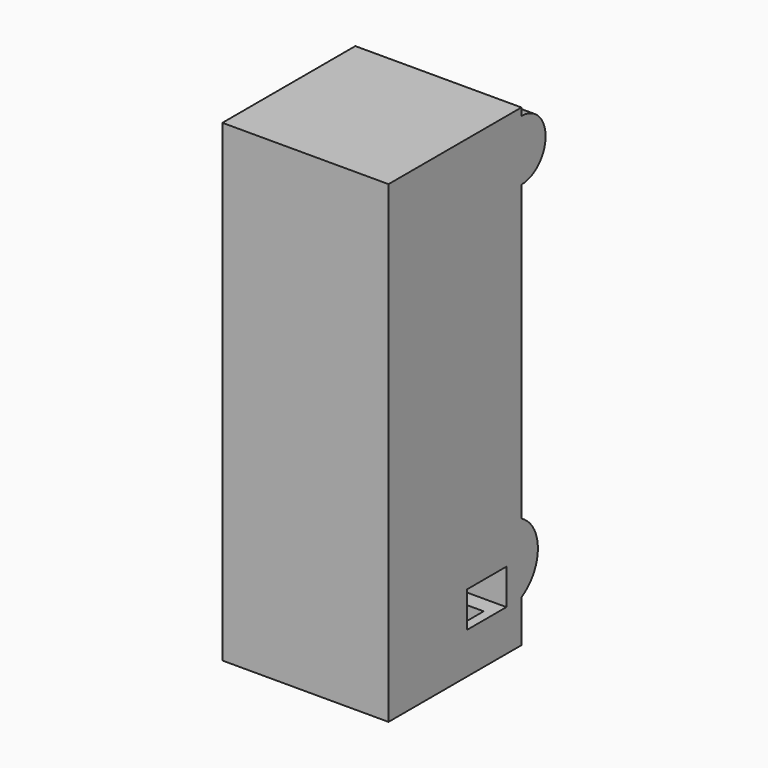
from build123d import *

# Parameters (mm, degrees)
F0_W        = 100
F0_H        = 100
F1_DEPTH    = 100
F2_W        = 88.9338813722
F2_H        = 88.2601328194
F3_DEPTH    = 90
F5_DEPTH    = 185
F6_T        = 5
F6_T3_DEPTH = 100
F6_T5_DEPTH = 98.2601328194
F6_T7_DEPTH = 98.9338813722
F7_W        = 90
F7_H        = 95
F8_DEPTH    = 8
F10_DEPTH   = 25
F11_R       = 23.6849070482
F11_R_2     = 18.1970048193
F12_DEPTH   = 25
F13_W       = 74.0287862718
F13_H       = 40.3192453086
F14_DEPTH   = 9
F15_W       = 33.1602711231
F15_H       = 63.8056004047
F16_DEPTH   = 25
F17_W       = 95
F17_H       = 277
F18_DEPTH   = 31
F19_W       = 29.5484475791
F19_H       = 21.4659199119
F20_DEPTH   = 25


# Not quite as in the source:
# - a shell that OpenCascade refuses in one call is made with other operations: the cavity is built on its own and cut out


with BuildPart() as f1:
    # F0 (on Front) → F1 (new body)
    with BuildSketch(Plane.XZ):
        with Locations((-6.5152887255, 3.7536189136)):
            Rectangle(F0_W, F0_H)
    extrude(amount=F1_DEPTH)

    # F2 (on face) → F3 (cut)
    with BuildSketch(Plane.XZ.offset(100)):
        with Locations((-6.6661592573, 4.4211242348)):
            Rectangle(F2_W, F2_H)
    extrude(amount=-F3_DEPTH, mode=Mode.SUBTRACT)

    # F4 (on face) → F5 (join)
    with BuildSketch(Plane.XY.offset(53.7536189136)):
        Polygon((-56.5152887255, -100), (43.4847112745, -100), (43.4847112745, -33.4126986563), (43.4847112745, 0), (-56.5152887255, 0), align=None)
    extrude(amount=F5_DEPTH)

    # F6: shell of thickness 5, made by hand


with BuildPart() as f6_core1:
    # F6_t2: copy of F1
    add(f1.part)

    # the walls: a layer under each face that stays
    f6_faces = [f6_core1.faces().sort_by_distance(p)[0] for p in [
        (43.4847112745, -50, 96.2536189136),
        (-6.5152887255, 0, 96.2536189136),
        (-56.5152887255, -50, 96.2536189136),
        (-51.1330999434, -55, 4.4211242348),
        (-6.6661592573, -10, 4.4211242348),
        (-6.6661592573, -55, -39.7089421749),
        (37.8007814288, -55, 4.4211242348),
        (-6.6661592573, -55, 48.5511906445),
        (-6.5152887255, -50, -46.2463810864),
    ]]
    thicken(f6_faces, amount=-F6_T, mode=Mode.SUBTRACT)

    # F6_s4 → F6_t3 (cut)
    with BuildSketch(Plane.XZ.offset(5)):
        Polygon((-51.0830999434, 48.5011906445), (-56.1330999434, 48.5511906445), (-56.1330999434, 53.5511906445), (-51.1330999434, 53.5511906445), align=None)
        Polygon((-51.0830999434, -39.6589421749), (-56.1330999434, -39.7089421749), (-56.1330999434, -44.7089421749), (-51.1330999434, -44.7089421749), align=None)
        Polygon((37.7507814288, -39.6589421749), (37.8007814288, -44.7089421749), (42.8007814288, -44.7089421749), (42.8007814288, -39.7089421749), align=None)
        Polygon((37.7507814288, 48.5011906445), (42.8007814288, 48.5511906445), (42.8007814288, 53.5511906445), (37.8007814288, 53.5511906445), align=None)
    extrude(amount=F6_T3_DEPTH, mode=Mode.SUBTRACT)

    # F6_s6 → F6_t5 (cut)
    with BuildSketch(Plane.XY.offset(-44.7089421749)):
        Polygon((-51.0830999434, -10.05), (-56.1330999434, -10), (-56.1330999434, -5), (-51.1330999434, -5), align=None)
        Polygon((37.7507814288, -10.05), (37.8007814288, -5), (42.8007814288, -5), (42.8007814288, -10), align=None)
    extrude(amount=F6_T5_DEPTH, mode=Mode.SUBTRACT)

    # F6_s8 → F6_t7 (cut)
    with BuildSketch(Plane.YZ.offset(-56.1330999434)):
        Polygon((-10.05, 48.5011906445), (-5, 48.5511906445), (-5, 53.5511906445), (-10, 53.5511906445), align=None)
        Polygon((-10.05, -39.6589421749), (-5, -39.7089421749), (-5, -44.7089421749), (-10, -44.7089421749), align=None)
    extrude(amount=F6_T7_DEPTH, mode=Mode.SUBTRACT)


with BuildPart() as f1_1:
    add(f1.part)

    # what is left inside the walls is the cavity
    f6_cavity = [f6_core1.part.solids().sort_by_distance(p)[0] for p in [
        (38.434711, -68.333333, 146.152405),
    ]]
    add(f6_cavity, mode=Mode.SUBTRACT)

    # F7 (on face) → F8 (join)
    with BuildSketch(Plane.XY.offset(238.7536189136)):
        with Locations((-6.5152887255, -52.5)):
            Rectangle(F7_W, F7_H)
    extrude(amount=-F8_DEPTH)

    # F9 (on face) → F10 (join)
    with BuildSketch(Plane(origin=(-56.5152887255, 0, 0), x_dir=(0, -1, 0), z_dir=(-1, 0, 0))):
        with BuildLine():
            ThreePointArc((0, 189.510354193), (12.2569085004, 194.5873319266), (17.333886234, 206.844240427))
            ThreePointArc((17.333886234, 206.844240427), (12.2569085004, 219.1011489274), (0, 224.178126661))
            Line((0, 224.178126661), (0, 189.510354193))
        make_face()
        with BuildLine():
            Line((0, 189.510354193), (0, 224.178126661))
            ThreePointArc((0, 224.178126661), (-17.333886234, 206.844240427), (0, 189.510354193))
        make_face()
        with BuildLine():
            Line((0, -23.6541135693), (0, 23.6541135693))
            ThreePointArc((0, 23.6541135693), (-15.7209434523, 0), (0, -23.6541135693))
        make_face()
    extrude(amount=-F10_DEPTH)

    # F11 (on face) → F12 (join)
    with BuildSketch(Plane.YZ.offset(43.4847112745)):
        with Locations((-11.2718828022, 0)):
            Circle(F11_R)
        with Locations((0, 216.0427719355)):
            Circle(F11_R_2)
    extrude(amount=-F12_DEPTH)

    # F13 (on face) → F14 (cut)
    with BuildSketch(Plane(origin=(0, 0, -46.2463810864), x_dir=(1, 0, 0), z_dir=(0, 0, -1))):
        with Locations((-6.1139781028, 59.594200924)):
            Rectangle(F13_W, F13_H)
    extrude(amount=-F14_DEPTH, mode=Mode.SUBTRACT)

    # F15 (on face) → F16 (cut)
    with BuildSketch(Plane(origin=(0, 0, 48.5511906445), x_dir=(1, 0, 0), z_dir=(0, 0, -1))):
        with Locations((9.9139763042, 41.9028002024)):
            Rectangle(F15_W, F15_H)
    extrude(amount=-F16_DEPTH, mode=Mode.SUBTRACT)

    # F17 (on face) → F18 (join)
    with BuildSketch(Plane.XZ.offset(100)):
        with Locations((-9.0152887255, 92.2536189136)):
            Rectangle(F17_W, F17_H)
    extrude(amount=-F18_DEPTH)

    # F19 (on face) → F20 (cut)
    with BuildSketch(Plane.YZ.offset(43.4847112745)):
        with Locations((-26.0461065918, -10.7329599559)):
            Rectangle(F19_W, F19_H)
    extrude(amount=-F20_DEPTH, mode=Mode.SUBTRACT)


solid = f1_1.part
